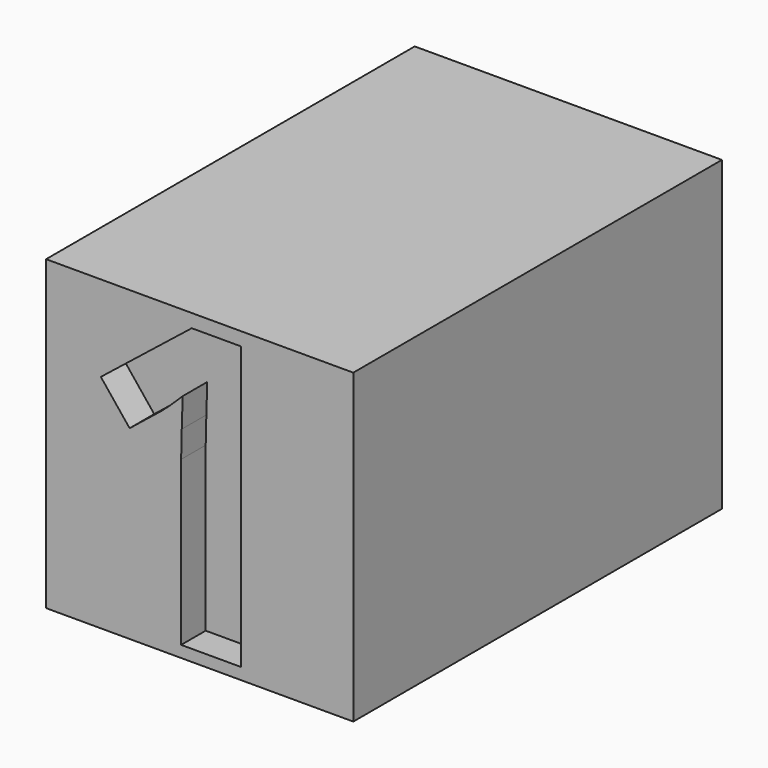
from build123d import *

# Parameters (mm, degrees)
F0_W         = 25.4
F0_H         = 25.4
F1_DEPTH     = 38.1
F2_TEXT_SIZE = 32.6877636124
F3_DEPTH     = 2.54


# Not quite as in the source:
# - Text() gives the source's letters only with a copy of the font that has no kerning and outlines rounded to 1/6400 em; it was checked with that copy


with BuildPart() as f1:
    # F0 (on Front) → F1 (new body)
    with BuildSketch(Plane.XZ):
        with Locations((12.7, 12.7)):
            Rectangle(F0_W, F0_H)
    extrude(amount=F1_DEPTH)

    # F2 (on face) → F3 (cut)
    with BuildSketch(Plane.XZ.offset(38.1)):
        with Locations((2.5962658692, 0.9565189248)):
            Text('1', F2_TEXT_SIZE, font='Open Sans', font_style=FontStyle.BOLD, text_align=(TextAlign.LEFT, TextAlign.BOTTOM))
    extrude(amount=-F3_DEPTH, mode=Mode.SUBTRACT)


solid = f1.part
